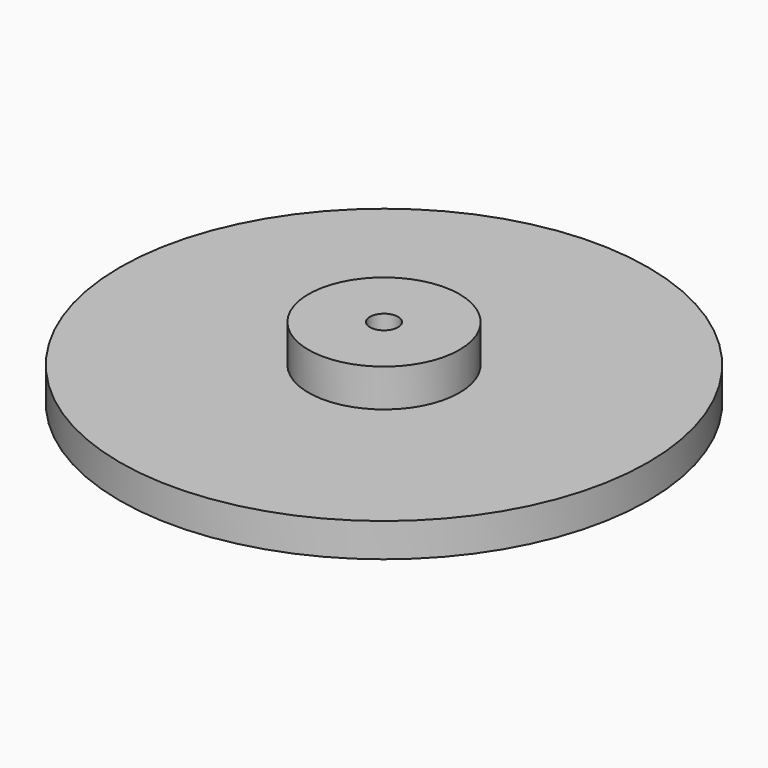
from build123d import *

# Parameters (mm, degrees)
F2_R     = 4.7625
F3_DEPTH = 9.525


# Not quite as in the source:
# - the program builds the solid bodies; features that only make, move or delete a surface that nothing else refers to are left out


with BuildPart() as f1:
    # F0 (on Front) → F1 (revolve)
    with BuildSketch(Plane.XZ):
        Polygon((0, 63.5), (0, 0), (88.9, 39.4620286852), (88.9, 50.8), (25.4, 50.8), (25.4, 63.5), align=None)
    revolve(axis=Axis((0, 0, 31.75), (0, 0, -1)))

    # F2 (on face) → F3 (cut)
    with BuildSketch(Plane.XY.offset(63.5)):
        Circle(F2_R)
    extrude(amount=-F3_DEPTH, mode=Mode.SUBTRACT)


solid = f1.part
